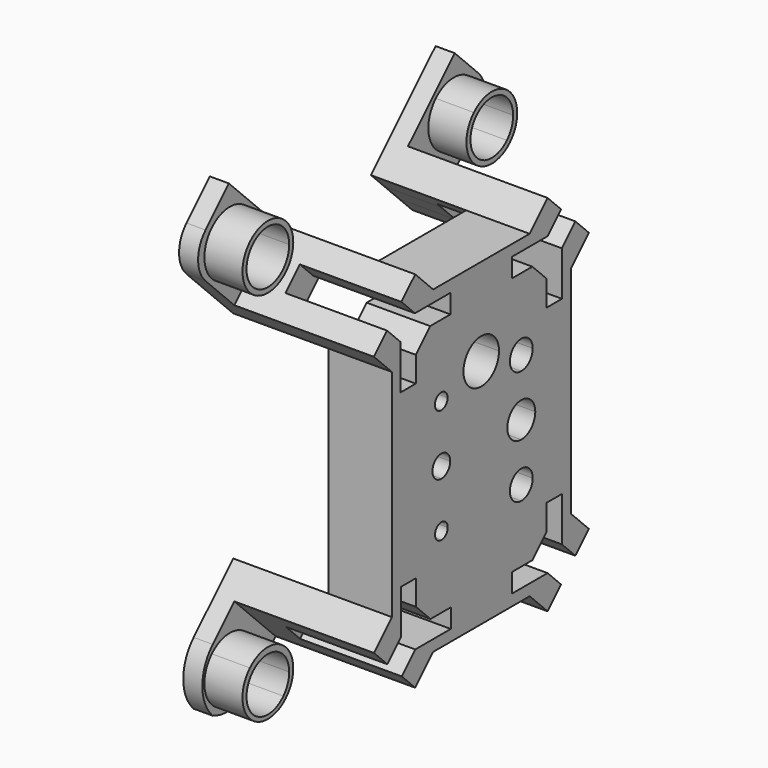
from build123d import *

# Parameters (mm, degrees)
F1_DEPTH     = 10
F2_W         = 25
F2_H         = 11.5
F3_DEPTH     = 5
F4_W         = 25
F4_H         = 11.5
F5_DEPTH     = 5
F6_W         = 25
F6_H         = 11.5
F7_DEPTH     = 5
F8_W         = 25
F8_H         = 11.5
F9_DEPTH     = 5
F10_W        = 16
F10_H        = 4
F11_DEPTH    = 8
F13_W        = 15
F13_H        = 11.5
F14_DEPTH    = 7
F15_DEPTH    = 10
F16_W        = 16
F16_H        = 4
F17_DEPTH    = 8
F18_W        = 15
F18_H        = 11.5
F19_DEPTH    = 7
F20_W        = 16
F20_H        = 4
F21_DEPTH    = 8
F22_W        = 16
F22_H        = 4
F23_DEPTH    = 8
F25_W        = 15
F25_H        = 11.5
F26_DEPTH    = 8
F27_W        = 15
F27_H        = 11.5
F28_DEPTH    = 8
F29_DEPTH    = 10
F30_DEPTH    = 6
F31_DEPTH    = 6
F32_DEPTH    = 6
F33_DEPTH    = 6
F34_DEPTH    = 25
F35_W        = 3
F35_H        = 11.5
F36_DEPTH    = 18
F38_DEPTH    = 6
F39_W        = 3
F39_H        = 11.5
F40_DEPTH    = 18
F42_DEPTH    = 6
F43_R        = 5
F44_R        = 5
F45_W        = 3
F45_H        = 11.5
F46_DEPTH    = 18
F48_DEPTH    = 6
F49_W        = 3
F49_H        = 11.5
F50_DEPTH    = 18
F52_DEPTH    = 6
F53_R        = 7
F55_DEPTH    = 25
F56_DEPTH    = 25
F57_DEPTH    = 25
F58_T1_DEPTH = 35.6917420766


# Not quite as in the source:
# - a fillet or chamfer that OpenCascade refuses, or shapes differently, is made with other operations: its cross-section is extruded or revolved along the edge and cut away or added
# - a feature names something its author has since deleted; it is built from what else it names


with BuildPart() as f1:
    # F0 (on Right) → F1 (new body)
    with BuildSketch(Plane.YZ):
        Polygon((2.6516504294, 44.6516504294), (0, 42), (0, 8), (8.1317279836, -0.1317279836), (27.1317304224, -0.1317279836), (29.7833808519, 2.5199224458), (32.6118079766, 5.3483495706), (35.2634584061, 8), (35.2634584061, 42), (32.6118079766, 44.6516504294), (29.7833808519, 47.4800775542), (27.1317304224, 50.1317279836), (8.1317279836, 50.1317279836), (5.4800775542, 47.4800775542), align=None)
    extrude(amount=F1_DEPTH)

    # F2 (on face) → F3 (join)
    with BuildSketch(Plane(origin=(0, 13.631729203, -13.631729203), x_dir=(-1, 0, 0), z_dir=(0, 0.7071067812, -0.7071067812))):
        with Locations((2.5, 24.8418848165)):
            Rectangle(F2_W, F2_H)
    extrude(amount=F3_DEPTH)

    # F4 (on face) → F5 (join)
    with BuildSketch(Plane(origin=(0, 38.631729203, 38.631729203), x_dir=(-1, 0, 0), z_dir=(0, 0.7071067812, 0.7071067812))):
        with Locations((2.5, 10.5134542428)):
            Rectangle(F4_W, F4_H)
    extrude(amount=F5_DEPTH)

    # F6 (on face) → F7 (join)
    with BuildSketch(Plane(origin=(0, 4, 4), x_dir=(1, 0, 0), z_dir=(0, -0.7071067812, -0.7071067812))):
        with Locations((-2.5, -0.0931457505)):
            Rectangle(F6_W, F6_H)
    extrude(amount=F7_DEPTH)

    # F8 (on face) → F9 (join)
    with BuildSketch(Plane(origin=(0, -21, 21), x_dir=(1, 0, 0), z_dir=(0, -0.7071067812, 0.7071067812))):
        with Locations((-2.5, 35.4484848098)):
            Rectangle(F8_W, F8_H)
    extrude(amount=F9_DEPTH)

    # F10 (on face) → F11 (cut)
    with BuildSketch(Plane(origin=(0, -24.5355339059, 24.5355339059), x_dir=(1, 0, 0), z_dir=(0, -0.7071067812, 0.7071067812))):
        with Locations((2, 35.3554848098)):
            Rectangle(F10_W, F10_H)
    extrude(amount=-F11_DEPTH, mode=Mode.SUBTRACT)

    # F13 (on face) → F14 (join)
    with BuildSketch(Plane(origin=(0, -21, 21), x_dir=(-1, 0, 0), z_dir=(0, 0.7071067812, -0.7071067812))):
        with Locations((7.5, 35.4484848098)):
            Rectangle(F13_W, F13_H)
    extrude(amount=F14_DEPTH)

    # F12 (on face) → F15 (cut)
    with BuildSketch(Plane.YZ.offset(10)):
        Polygon((4.5356369671, 48.29299628), (7.5356369671, 45.29299628), (11.5356369671, 45.29299628), (11.5356369671, 48.29299628), align=None)
        Polygon((4.7072098424, 38.4645691552), (4.7072098424, 42.4645691552), (1.7072098424, 45.4645691552), (1.7072098424, 38.4645691552), align=None)
    extrude(amount=-F15_DEPTH, mode=Mode.SUBTRACT)

    # F16 (on face) → F17 (cut)
    with BuildSketch(Plane(origin=(0, 42.167263109, 42.167263109), x_dir=(-1, 0, 0), z_dir=(0, 0.7071067812, 0.7071067812))):
        with Locations((-2, 10.5134542428)):
            Rectangle(F16_W, F16_H)
    extrude(amount=-F17_DEPTH, mode=Mode.SUBTRACT)

    # F18 (on face) → F19 (join)
    with BuildSketch(Plane(origin=(0, 38.631729203, 38.631729203), x_dir=(1, 0, 0), z_dir=(0, -0.7071067812, -0.7071067812))):
        with Locations((-7.5, 10.5134542428)):
            Rectangle(F18_W, F18_H)
    extrude(amount=F19_DEPTH)

    # F20 (on face) → F21 (cut)
    with BuildSketch(Plane(origin=(0, 17.167263109, -17.167263109), x_dir=(-1, 0, 0), z_dir=(0, 0.7071067812, -0.7071067812))):
        with Locations((-2, 24.8418848165)):
            Rectangle(F20_W, F20_H)
    extrude(amount=-F21_DEPTH, mode=Mode.SUBTRACT)

    # F22 (on face) → F23 (cut)
    with BuildSketch(Plane(origin=(0, 0.4644660941, 0.4644660941), x_dir=(1, 0, 0), z_dir=(0, -0.7071067812, -0.7071067812))):
        with Locations((2, -0.0931457505)):
            Rectangle(F22_W, F22_H)
    extrude(amount=-F23_DEPTH, mode=Mode.SUBTRACT)

    # F25 (on face) → F26 (join)
    with BuildSketch(Plane(origin=(0, 4, 4), x_dir=(-1, 0, 0), z_dir=(0, 0.7071067812, 0.7071067812))):
        with Locations((7.5, -0.0931457505)):
            Rectangle(F25_W, F25_H)
    extrude(amount=F26_DEPTH)

    # F27 (on face) → F28 (join)
    with BuildSketch(Plane(origin=(0, 13.631729203, -13.631729203), x_dir=(1, 0, 0), z_dir=(0, -0.7071067812, 0.7071067812))):
        with Locations((-7.5, 24.8418848165)):
            Rectangle(F27_W, F27_H)
    extrude(amount=F28_DEPTH)

    # F24 (on face) → F29 (cut)
    with BuildSketch(Plane.YZ.offset(10)):
        Polygon((30.4904876331, 11.4696699141), (30.4904876331, 7.4696699141), (33.4904876331, 4.4696699141), (33.4904876331, 11.4696699141), align=None)
        Polygon((23.6620605083, 1.6412427894), (30.6620605083, 1.6412427894), (27.6620605083, 4.6412427894), (23.6620605083, 4.6412427894), align=None)
        Polygon((1.772970773, 4.4696699141), (4.772970773, 7.4696699141), (4.772970773, 11.4696699141), (1.772970773, 11.4696699141), align=None)
        Polygon((11.6013978978, 4.6412427894), (7.6013978978, 4.6412427894), (4.6013978978, 1.6412427894), (11.6013978978, 1.6412427894), align=None)
        Polygon((33.4904876331, 38.5303300859), (33.4904876331, 45.5303300859), (30.4904876331, 42.5303300859), (30.4904876331, 38.5303300859), align=None)
        Polygon((23.6620605083, 45.3587572106), (27.6620605083, 45.3587572106), (30.6620605083, 48.3587572106), (23.6620605083, 48.3587572106), align=None)
    extrude(amount=-F29_DEPTH, mode=Mode.SUBTRACT)

    # F30 (cut): a face of the model
    f30_faces = [f1.faces().sort_by_distance(p)[0] for p in [
        (0, 29.5906779781, 5.5410524444),
    ]]
    extrude(f30_faces, amount=-F30_DEPTH, mode=Mode.SUBTRACT)

    # F31 (cut): a face of the model
    f31_faces = [f1.faces().sort_by_distance(p)[0] for p in [
        (0, 29.5906779781, 44.4589475556),
    ]]
    extrude(f31_faces, amount=-F31_DEPTH, mode=Mode.SUBTRACT)

    # F32 (cut): a face of the model
    f32_faces = [f1.faces().sort_by_distance(p)[0] for p in [
        (0, 5.649683327, 44.4366839714),
    ]]
    extrude(f32_faces, amount=-F32_DEPTH, mode=Mode.SUBTRACT)

    # F33 (cut): a face of the model
    f33_faces = [f1.faces().sort_by_distance(p)[0] for p in [
        (0, 5.672780428, 5.5410524444),
    ]]
    extrude(f33_faces, amount=-F33_DEPTH, mode=Mode.SUBTRACT)

    # F0 (on Right) → F34 (cut)
    with BuildSketch(Plane.YZ):
        Polygon((2.6516504294, 44.6516504294), (0, 42), (0, 8), (8.1317279836, -0.1317279836), (27.1317304224, -0.1317279836), (29.7833808519, 2.5199224458), (32.6118079766, 5.3483495706), (35.2634584061, 8), (35.2634584061, 42), (32.6118079766, 44.6516504294), (29.7833808519, 47.4800775542), (27.1317304224, 50.1317279836), (8.1317279836, 50.1317279836), (5.4800775542, 47.4800775542), align=None)
    extrude(amount=-F34_DEPTH, mode=Mode.SUBTRACT)

    # F35 (on face) → F36 (join)
    with BuildSketch(Plane(origin=(0, 38.631729203, 38.631729203), x_dir=(1, 0, 0), z_dir=(0, -0.7071067812, -0.7071067812))):
        with Locations((-13.5, 10.5134542428)):
            Rectangle(F35_W, F35_H)
    extrude(amount=-F36_DEPTH)

    # F37 (on face) → F38 (join)
    with BuildSketch(Plane.YZ.offset(-12)):
        with BuildLine():
            ThreePointArc((36.1473418826, 58.086679272), (36.1473418826, 51.0156114601), (43.2184096944, 51.0156114601))
            Line((43.2184096944, 51.0156114601), (42.6527242695, 51.5812968851))
            ThreePointArc((42.6527242695, 51.5812968851), (36.7130273075, 51.5812968851), (36.7130273075, 57.520993847))
            Line((36.7130273075, 57.520993847), (36.1473418826, 58.086679272))
        make_face()
        with BuildLine():
            Line((42.6527242695, 51.5812968851), (43.2184096944, 51.0156114601))
            ThreePointArc((43.2184096944, 51.0156114601), (44.3022734511, 52.6377282042), (44.6828757885, 54.5511453661))
            ThreePointArc((44.6828757885, 54.5511453661), (41.5962929503, 59.1705430286), (36.1473418826, 58.086679272))
            Line((36.1473418826, 58.086679272), (36.7130273075, 57.520993847))
            ThreePointArc((36.7130273075, 57.520993847), (41.2901462044, 58.4314394026), (43.8828757885, 54.5511453661))
            ThreePointArc((43.8828757885, 54.5511453661), (43.5631698251, 52.9438749501), (42.6527242695, 51.5812968851))
        make_face()
    extrude(amount=F38_DEPTH)

    # F39 (on face) → F40 (join)
    with BuildSketch(Plane(origin=(0, -21, 21), x_dir=(-1, 0, 0), z_dir=(0, 0.7071067812, -0.7071067812))):
        with Locations((13.5, 35.4484848098)):
            Rectangle(F39_W, F39_H)
    extrude(amount=-F40_DEPTH)

    # F41 (on face) → F42 (join)
    with BuildSketch(Plane.YZ.offset(-12)):
        with BuildLine():
            Line((-1.4495689014, 57.520993847), (-0.8838834765, 58.086679272))
            ThreePointArc((-0.8838834765, 58.086679272), (-7.9549512883, 58.086679272), (-7.9549512883, 51.0156114601))
            Line((-7.9549512883, 51.0156114601), (-7.3892658634, 51.5812968851))
            ThreePointArc((-7.3892658634, 51.5812968851), (-7.3892658634, 57.520993847), (-1.4495689014, 57.520993847))
        make_face()
        with BuildLine():
            ThreePointArc((0.5805826176, 54.5511453661), (0.1999802801, 56.4645625279), (-0.8838834765, 58.086679272))
            Line((-0.8838834765, 58.086679272), (-1.4495689014, 57.520993847))
            ThreePointArc((-1.4495689014, 57.520993847), (-0.5391233459, 56.158415782), (-0.2194173824, 54.5511453661))
            ThreePointArc((-0.2194173824, 54.5511453661), (-2.8121469665, 50.6708513295), (-7.3892658634, 51.5812968851))
            Line((-7.3892658634, 51.5812968851), (-7.9549512883, 51.0156114601))
            ThreePointArc((-7.9549512883, 51.0156114601), (-2.5060002206, 49.9317477035), (0.5805826176, 54.5511453661))
        make_face()
    extrude(amount=F42_DEPTH)

    # F43
    f43_edges = [f1.edges().sort_by_distance(p)[0] for p in [
        (-13.5, -12.727922, 54.727922),
    ]]
    fillet(f43_edges, radius=F43_R)

    # F44
    f44_edges = [f1.edges().sort_by_distance(p)[0] for p in [
        (-13.5, 47.99138, 54.727922),
    ]]
    fillet(f44_edges, radius=F44_R)

    # F45 (on face) → F46 (join)
    with BuildSketch(Plane(origin=(0, 13.631729203, -13.631729203), x_dir=(1, 0, 0), z_dir=(0, -0.7071067812, 0.7071067812))):
        with Locations((-13.5, 24.8418848165)):
            Rectangle(F45_W, F45_H)
    extrude(amount=-F46_DEPTH)

    # F47 (on face) → F48 (join)
    with BuildSketch(Plane.YZ.offset(-12)):
        with BuildLine():
            Line((42.6527242695, -1.5812968851), (43.2184096944, -1.0156114601))
            ThreePointArc((43.2184096944, -1.0156114601), (36.1473418826, -1.0156114601), (36.1473418826, -8.086679272))
            Line((36.1473418826, -8.086679272), (36.7130273075, -7.520993847))
            ThreePointArc((36.7130273075, -7.520993847), (36.7130273075, -1.5812968851), (42.6527242695, -1.5812968851))
        make_face()
        with BuildLine():
            ThreePointArc((44.6828757885, -4.5511453661), (44.3022734511, -2.6377282042), (43.2184096944, -1.0156114601))
            Line((43.2184096944, -1.0156114601), (42.6527242695, -1.5812968851))
            ThreePointArc((42.6527242695, -1.5812968851), (43.5631698251, -2.9438749501), (43.8828757885, -4.5511453661))
            ThreePointArc((43.8828757885, -4.5511453661), (41.2901462044, -8.4314394026), (36.7130273075, -7.520993847))
            Line((36.7130273075, -7.520993847), (36.1473418826, -8.086679272))
            ThreePointArc((36.1473418826, -8.086679272), (41.5962929503, -9.1705430286), (44.6828757885, -4.5511453661))
        make_face()
    extrude(amount=F48_DEPTH)

    # F49 (on face) → F50 (join)
    with BuildSketch(Plane(origin=(0, 4, 4), x_dir=(-1, 0, 0), z_dir=(0, 0.7071067812, 0.7071067812))):
        with Locations((13.5, -0.0931457505)):
            Rectangle(F49_W, F49_H)
    extrude(amount=-F50_DEPTH)

    # F51 (on face) → F52 (join)
    with BuildSketch(Plane.YZ.offset(-12)):
        with BuildLine():
            Line((-1.362496148, -7.6080666005), (-0.8838834765, -8.086679272))
            ThreePointArc((-0.8838834765, -8.086679272), (0.1999802801, -6.4645625279), (0.5805826176, -4.5511453661))
            ThreePointArc((0.5805826176, -4.5511453661), (-2.5060002206, 0.0682522965), (-7.9549512883, -1.0156114601))
            Line((-7.9549512883, -1.0156114601), (-7.2995619216, -1.6710008269))
            ThreePointArc((-7.2995619216, -1.6710008269), (-2.7545761084, -0.871978139), (-0.2194173824, -4.7279220614))
            ThreePointArc((-0.2194173824, -4.7279220614), (-0.5156327326, -6.2772656022), (-1.362496148, -7.6080666005))
        make_face()
        with BuildLine():
            ThreePointArc((-7.9549512883, -1.0156114601), (-7.9549512883, -8.086679272), (-0.8838834765, -8.086679272))
            Line((-0.8838834765, -8.086679272), (-1.362496148, -7.6080666005))
            ThreePointArc((-1.362496148, -7.6080666005), (-7.3892658634, -7.6977705423), (-7.2995619216, -1.6710008269))
            Line((-7.2995619216, -1.6710008269), (-7.9549512883, -1.0156114601))
        make_face()
    extrude(amount=F52_DEPTH)

    # F53
    f53_edges = [f1.edges().sort_by_distance(p)[0] for p in [
        (-13.5, -12.727922, -4.727922),
        (-13.5, 47.99138, -4.727922),
    ]]
    fillet(f53_edges, radius=F53_R)

    # F54 (on face) → F55 (cut)
    with BuildSketch(Plane.YZ.offset(10)):
        with BuildLine():
            Line((25.4904876331, 27.75), (25.4904876331, 22.25))
            ThreePointArc((25.4904876331, 22.25), (27.4350312813, 23.0554563517), (28.2404876331, 25))
            ThreePointArc((28.2404876331, 25), (27.4350312813, 26.9445436483), (25.4904876331, 27.75))
        make_face()
        with BuildLine():
            ThreePointArc((25.4904876331, 27.75), (22.7404876331, 25), (25.4904876331, 22.25))
            Line((25.4904876331, 22.25), (25.4904876331, 27.75))
        make_face()
    extrude(amount=-F55_DEPTH, mode=Mode.SUBTRACT)

    # F54 (on face) → F56 (cut)
    with BuildSketch(Plane.YZ.offset(10)):
        with BuildLine():
            ThreePointArc((25.4904876331, 36.25), (23.2404876331, 34), (25.4904876331, 31.75))
            Line((25.4904876331, 31.75), (25.4904876331, 36.25))
        make_face()
        with BuildLine():
            Line((25.4904876331, 36.25), (25.4904876331, 31.75))
            ThreePointArc((25.4904876331, 31.75), (27.0814778907, 32.4090097423), (27.7404876331, 34))
            ThreePointArc((27.7404876331, 34), (27.0814778907, 35.5909902577), (25.4904876331, 36.25))
        make_face()
        with BuildLine():
            ThreePointArc((25.4904876331, 18.25), (23.2404876331, 16), (25.4904876331, 13.75))
            Line((25.4904876331, 13.75), (25.4904876331, 18.25))
        make_face()
        with BuildLine():
            Line((25.4904876331, 18.25), (25.4904876331, 13.75))
            ThreePointArc((25.4904876331, 13.75), (27.0814778907, 14.4090097423), (27.7404876331, 16))
            ThreePointArc((27.7404876331, 16), (27.0814778907, 17.5909902577), (25.4904876331, 18.25))
        make_face()
    extrude(amount=-F56_DEPTH, mode=Mode.SUBTRACT)

    # F54 (on face) → F57 (cut)
    with BuildSketch(Plane.YZ.offset(10)):
        with BuildLine():
            ThreePointArc((25.4904876331, 18.25), (23.2404876331, 16), (25.4904876331, 13.75))
            Line((25.4904876331, 13.75), (25.4904876331, 18.25))
        make_face()
        with BuildLine():
            ThreePointArc((25.4904876331, 36.25), (23.2404876331, 34), (25.4904876331, 31.75))
            Line((25.4904876331, 31.75), (25.4904876331, 36.25))
        make_face()
        with BuildLine():
            Line((25.4904876331, 36.25), (25.4904876331, 31.75))
            ThreePointArc((25.4904876331, 31.75), (27.0814778907, 32.4090097423), (27.7404876331, 34))
            ThreePointArc((27.7404876331, 34), (27.0814778907, 35.5909902577), (25.4904876331, 36.25))
        make_face()
        with BuildLine():
            ThreePointArc((25.4904876331, 27.75), (22.7404876331, 25), (25.4904876331, 22.25))
            Line((25.4904876331, 22.25), (25.4904876331, 27.75))
        make_face()
        with BuildLine():
            Line((25.4904876331, 27.75), (25.4904876331, 22.25))
            ThreePointArc((25.4904876331, 22.25), (27.4350312813, 23.0554563517), (28.2404876331, 25))
            ThreePointArc((28.2404876331, 25), (27.4350312813, 26.9445436483), (25.4904876331, 27.75))
        make_face()
        with BuildLine():
            Line((25.4904876331, 18.25), (25.4904876331, 13.75))
            ThreePointArc((25.4904876331, 13.75), (27.0814778907, 14.4090097423), (27.7404876331, 16))
            ThreePointArc((27.7404876331, 16), (27.0814778907, 17.5909902577), (25.4904876331, 18.25))
        make_face()
        with BuildLine():
            ThreePointArc((9.7526272163, 17.2171178992), (8.5046509308, 15.9650974557), (9.7566713743, 14.7171211702))
            Line((9.7566713743, 14.7171211702), (9.7526272163, 17.2171178992))
        make_face()
        with BuildLine():
            ThreePointArc((9.7235092411, 35.2171178992), (8.4755329556, 33.9650974557), (9.727553399, 32.7171211702))
            Line((9.727553399, 32.7171211702), (9.7235092411, 35.2171178992))
        make_face()
        with BuildLine():
            Line((9.7235092411, 35.2171178992), (9.727553399, 32.7171211702))
            ThreePointArc((9.727553399, 32.7171211702), (10.6101294205, 33.0839512604), (10.9755313201, 33.9671195347))
            ThreePointArc((10.9755313201, 33.9671195347), (10.6086995943, 34.8517176351), (9.7235092411, 35.2171178992))
        make_face()
        with BuildLine():
            ThreePointArc((9.7372593971, 26.7171172449), (7.9900925974, 24.9642886241), (9.7429212182, 23.2171218244))
            Line((9.7429212182, 23.2171218244), (9.7372593971, 26.7171172449))
        make_face()
        with BuildLine():
            Line((9.7372593971, 26.7171172449), (9.7429212182, 23.2171218244))
            ThreePointArc((9.7429212182, 23.2171218244), (10.9785276483, 23.7306839507), (11.4900903077, 24.9671195347))
            ThreePointArc((11.4900903077, 24.9671195347), (10.9765258916, 26.2055568753), (9.7372593971, 26.7171172449))
        make_face()
        with BuildLine():
            Line((9.7526272163, 17.2171178992), (9.7566713743, 14.7171211702))
            ThreePointArc((9.7566713743, 14.7171211702), (10.6392473958, 15.0839512604), (11.0046492953, 15.9671195347))
            ThreePointArc((11.0046492953, 15.9671195347), (10.6378175696, 16.8517176351), (9.7526272163, 17.2171178992))
        make_face()
        with BuildLine():
            ThreePointArc((17.5988487377, 39.8258767453), (15.1239750036, 33.8510030112), (21.0988487377, 36.3258767453))
            ThreePointArc((21.0988487377, 36.3258767453), (20.0737224719, 38.8007504795), (17.5988487377, 39.8258767453))
        make_face()
    extrude(amount=-F57_DEPTH, mode=Mode.SUBTRACT)

    # F58: fillet of radius 7 on 2 edges, made by hand

    # F58_s2 → F58_t1 (cut)
    with BuildSketch(Plane.YZ.offset(-31.3458710383)):
        with BuildLine():
            ThreePointArc((-7.7781745931, -9.6776695297), (-3.6514974763, -10.1702117221), (0.0271164245, -8.2363395428))
            Line((0.0271164245, -8.2363395428), (-4.5961940777, -12.859650045))
            Line((-4.5961940777, -12.859650045), (-7.7781745931, -9.6776695297))
        make_face()
        with BuildLine():
            ThreePointArc((35.2363419816, -8.2363395428), (38.9149558824, -10.1702117221), (43.0416329991, -9.6776695297))
            Line((43.0416329991, -9.6776695297), (39.8596524838, -12.859650045))
            Line((39.8596524838, -12.859650045), (35.2363419816, -8.2363395428))
        make_face()
    extrude(amount=F58_T1_DEPTH, mode=Mode.SUBTRACT)


solid = f1.part
